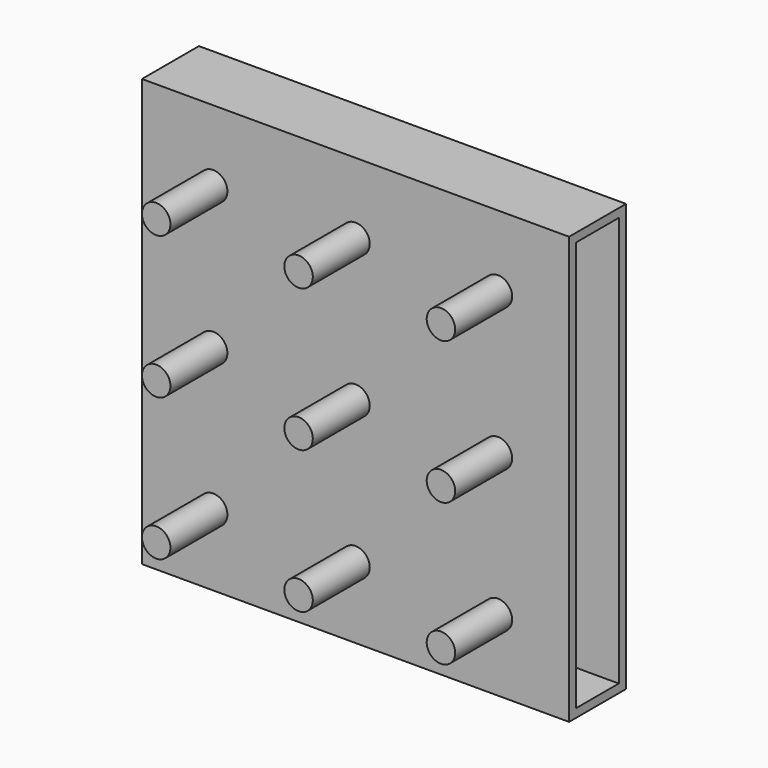
from build123d import *

# Parameters (mm, degrees)
F0_R     = 2.54
F1_DEPTH = 25.4
F0_W     = 25.4
F0_H     = 25.4
F2_DEPTH = 12.7
F3_W     = 9.5477323048
F3_H     = 73.1356367469
F4_DEPTH = 71.12


with BuildPart() as f1:
    # F0 (on Front) → F1 (new body)
    with BuildSketch(Plane.XZ):
        with Locations((-31.5060045898, 27.5050493181)):
            Circle(F0_R)
    extrude(amount=F1_DEPTH)


with BuildPart() as f1b:
    # F0 (on Front) → F1, piece 2 (new body)
    with BuildSketch(Plane.XZ):
        with Locations((-6.1060045898, 27.5050493181)):
            Circle(F0_R)
    extrude(amount=F1_DEPTH)


with BuildPart() as f1c:
    # F0 (on Front) → F1, piece 3 (new body)
    with BuildSketch(Plane.XZ):
        with Locations((19.2939954102, 27.5050493181)):
            Circle(F0_R)
    extrude(amount=F1_DEPTH)


with BuildPart() as f1d:
    # F0 (on Front) → F1, piece 4 (new body)
    with BuildSketch(Plane.XZ):
        with Locations((-31.5060045898, 2.1050493181)):
            Circle(F0_R)
    extrude(amount=F1_DEPTH)


with BuildPart() as f1e:
    # F0 (on Front) → F1, piece 5 (new body)
    with BuildSketch(Plane.XZ):
        with Locations((-6.1060045898, 2.1050493181)):
            Circle(F0_R)
    extrude(amount=F1_DEPTH)


with BuildPart() as f1f:
    # F0 (on Front) → F1, piece 6 (new body)
    with BuildSketch(Plane.XZ):
        with Locations((19.2939954102, 2.1050493181)):
            Circle(F0_R)
    extrude(amount=F1_DEPTH)


with BuildPart() as f1g:
    # F0 (on Front) → F1, piece 7 (new body)
    with BuildSketch(Plane.XZ):
        with Locations((-31.5060045898, -23.2949506819)):
            Circle(F0_R)
    extrude(amount=F1_DEPTH)


with BuildPart() as f1h:
    # F0 (on Front) → F1, piece 8 (new body)
    with BuildSketch(Plane.XZ):
        with Locations((-6.1060045898, -23.2949506819)):
            Circle(F0_R)
    extrude(amount=F1_DEPTH)


with BuildPart() as f1i:
    # F0 (on Front) → F1, piece 9 (new body)
    with BuildSketch(Plane.XZ):
        with Locations((19.2939954102, -23.2949506819)):
            Circle(F0_R)
    extrude(amount=F1_DEPTH)


with BuildPart() as f2:
    # F0 (on Front) → F2 (new body)
    with BuildSketch(Plane.XZ):
        Polygon((-18.8060045898, 40.2050493181), (-44.2060045898, 40.2050493181), (-44.2060045898, 14.8050493181), (-40.7688207924, 14.8050493181), (-18.8060045898, 14.8050493181), align=None)
        with Locations((-31.5060045898, 27.5050493181)):
            Circle(F0_R, mode=Mode.SUBTRACT)
        Polygon((-40.7688207924, 14.8050493181), (-44.2060045898, 14.8050493181), (-44.2060045898, -10.5949506819), (-18.8060045898, -10.5949506819), (-18.8060045898, 14.8050493181), align=None)
        with Locations((-31.5060045898, 2.1050493181)):
            Circle(F0_R, mode=Mode.SUBTRACT)
        with Locations((-6.1060045898, 27.5050493181)):
            Rectangle(F0_W, F0_H)
        with Locations((-6.1060045898, 27.5050493181)):
            Circle(F0_R, mode=Mode.SUBTRACT)
        with Locations((-31.5060045898, -23.2949506819)):
            Rectangle(F0_W, F0_H)
        with Locations((-31.5060045898, -23.2949506819)):
            Circle(F0_R, mode=Mode.SUBTRACT)
        with Locations((19.2939954102, 27.5050493181)):
            Rectangle(F0_W, F0_H)
        with Locations((19.2939954102, 27.5050493181)):
            Circle(F0_R, mode=Mode.SUBTRACT)
        with Locations((-6.1060045898, -23.2949506819)):
            Rectangle(F0_W, F0_H)
        with Locations((-6.1060045898, -23.2949506819)):
            Circle(F0_R, mode=Mode.SUBTRACT)
        with Locations((19.2939954102, 2.1050493181)):
            Rectangle(F0_W, F0_H)
        with Locations((19.2939954102, 2.1050493181)):
            Circle(F0_R, mode=Mode.SUBTRACT)
        with Locations((19.2939954102, -23.2949506819)):
            Rectangle(F0_W, F0_H)
        with Locations((19.2939954102, -23.2949506819)):
            Circle(F0_R, mode=Mode.SUBTRACT)
        with Locations((-6.1060045898, 2.1050493181)):
            Rectangle(F0_W, F0_H)
        with Locations((-6.1060045898, 2.1050493181)):
            Circle(F0_R, mode=Mode.SUBTRACT)
    extrude(amount=F2_DEPTH)

    # F3 (on face) → F4 (cut)
    with BuildSketch(Plane.YZ.offset(31.9939954102)):
        with Locations((-6.396981189, 2.1005012095)):
            Rectangle(F3_W, F3_H)
    extrude(amount=-F4_DEPTH, mode=Mode.SUBTRACT)


solid = Compound([f1.part, f1b.part, f1c.part, f1d.part, f1e.part, f1f.part, f1g.part, f1h.part, f1i.part, f2.part])
